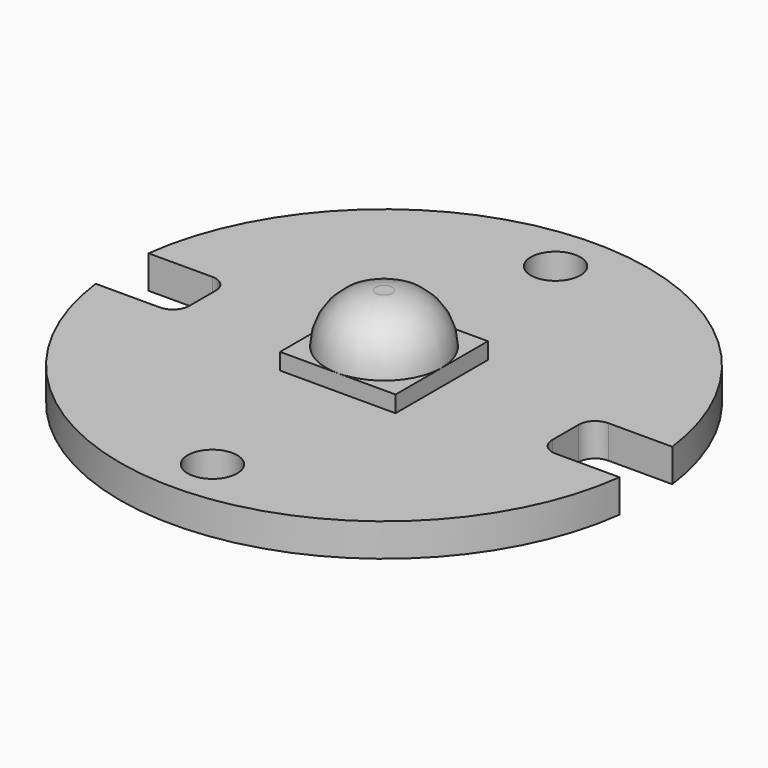
from build123d import *

# Parameters (mm, degrees)
F0_R     = 16
F1_DEPTH = 2
F2_R     = 1.5
F3_DEPTH = 2.001
F4_W     = 7
F4_H     = 7
F5_DEPTH = 1
F7_DEPTH = 3


# Not quite as in the source:
# - a fillet or chamfer that OpenCascade refuses, or shapes differently, is made with other operations: its cross-section is extruded or revolved along the edge and cut away or added


with BuildPart() as f1:
    # F0 (on Top) → F1 (new body)
    with BuildSketch(Plane.XY):
        Circle(F0_R)
    extrude(amount=F1_DEPTH)

    # F2 (on face) → F3 (cut, through all)
    with BuildSketch(Plane.XY.offset(2)):
        with BuildLine():
            ThreePointArc((-11, 1), (-11.2928932188, 1.7071067812), (-12, 2))
            Line((-12, 2), (-15.8745078664, 2))
            ThreePointArc((-15.8745078664, 2), (-16, 0), (-15.8745078664, -2))
            Line((-15.8745078664, -2), (-12, -2))
            ThreePointArc((-12, -2), (-11.2928932188, -1.7071067812), (-11, -1))
            Line((-11, -1), (-11, 1))
        make_face()
        with BuildLine():
            ThreePointArc((-15.8745078664, -2), (-16, 0), (-15.8745078664, 2))
            Line((-15.8745078664, 2), (-21, 2))
            Line((-21, 2), (-21, -2))
            Line((-21, -2), (-15.8745078664, -2))
        make_face()
        with BuildLine():
            ThreePointArc((16, 0), (15.9685961478, 1.0019666007), (15.8745078664, 2))
            Line((15.8745078664, 2), (12, 2))
            ThreePointArc((12, 2), (11.2928932188, 1.7071067812), (11, 1))
            Line((11, 1), (11, -1))
            ThreePointArc((11, -1), (11.2928932188, -1.7071067812), (12, -2))
            Line((12, -2), (15.8745078664, -2))
            ThreePointArc((15.8745078664, -2), (15.9685961478, -1.0019666007), (16, 0))
        make_face()
        with BuildLine():
            Line((21, 2), (15.8745078664, 2))
            ThreePointArc((15.8745078664, 2), (15.9685961478, 1.0019666007), (16, 0))
            ThreePointArc((16, 0), (15.9685961478, -1.0019666007), (15.8745078664, -2))
            Line((15.8745078664, -2), (21, -2))
            Line((21, -2), (21, 2))
        make_face()
        with Locations((0, 13)):
            Circle(F2_R)
        with Locations((0, -13)):
            Circle(F2_R)
    extrude(amount=-F3_DEPTH, mode=Mode.SUBTRACT)


with BuildPart() as f5:
    # F4 (on face) → F5 (new body)
    with BuildSketch(Plane.XY.offset(2)):
        Rectangle(F4_W, F4_H)
    extrude(amount=F5_DEPTH)


with BuildPart() as f7:
    # F6 (on face) → F7 (new body)
    with BuildSketch(Plane.XY.offset(3)):
        with BuildLine():
            ThreePointArc((0, -3.5), (2.4748737342, -2.4748737342), (3.5, 0))
            ThreePointArc((3.5, 0), (2.4748737342, 2.4748737342), (0, 3.5))
            ThreePointArc((0, 3.5), (-2.4748737342, 2.4748737342), (-3.5, 0))
            ThreePointArc((-3.5, 0), (-2.4748737342, -2.4748737342), (0, -3.5))
        make_face()
    extrude(amount=F7_DEPTH)

    # F8: fillet of radius 3 on 1 edges, made by hand

    # F8_s1 → F8_t2 (revolve, cut)
    with BuildSketch(Plane.YZ):
        with BuildLine():
            ThreePointArc((3.5, 3), (2.6213203436, 5.1213203436), (0.5, 6))
            Line((0.5, 6), (3.5, 6))
            Line((3.5, 6), (3.5, 3))
        make_face()
    revolve(axis=Axis((0, 0, 6), (0, 0, -1)), mode=Mode.SUBTRACT)


solid = Compound([f1.part, f5.part, f7.part])
